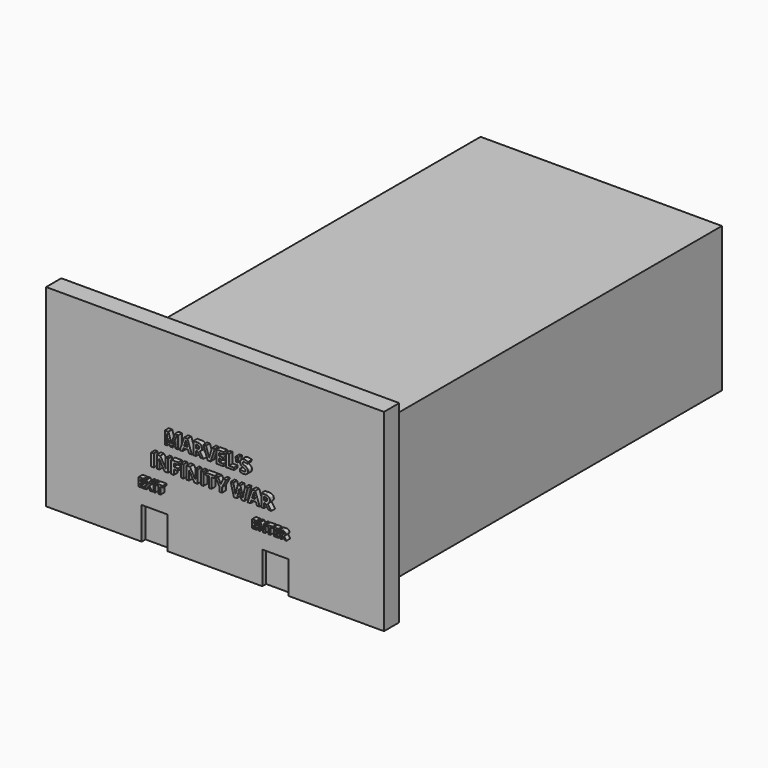
from build123d import *

# Parameters (mm, degrees)
F0_W          = 15240
F0_H          = 9144
F1_DEPTH      = 30480
F2_W          = 15240
F2_H          = 1203.030090332
F3_DEPTH      = 3048
F4_W          = 822.96
F4_H          = 2042.16
F5_DEPTH      = 304.8
F7_TEXT_SIZE  = 751.4417171478
F8_DEPTH      = 304.8
F9_TEXT_SIZE  = 701.0988429122
F10_DEPTH     = 304.8
F12_DEPTH     = 3048
F14_DEPTH     = 3048
F15_TEXT_SIZE = 1106.0376962026
F16_DEPTH     = 304.8


# Not quite as in the source:
# - Text() gives the source's letters only with a copy of the font that has no kerning and outlines rounded to 1/6400 em; it was checked with that copy


with BuildPart() as f1:
    # F0 (on Front) → F1 (new body)
    with BuildSketch(Plane.XZ):
        with Locations((7566.6301758587, 4516.3960119644)):
            Rectangle(F0_W, F0_H)
    extrude(amount=F1_DEPTH)

    # F2 (on face) → F3 (join)
    with BuildSketch(Plane.XY.offset(9088.3960119644)):
        with Locations((7566.6301758587, -29878.484954834)):
            Rectangle(F2_W, F2_H)
    extrude(amount=F3_DEPTH)

    # F4 (on face) → F5 (cut)
    with BuildSketch(Plane.XZ.offset(30480)):
        with Locations((3345.1501758587, 965.4760119644)):
            Rectangle(F4_W, F4_H)
        with Locations((4168.1101758587, 965.4760119644)):
            Rectangle(F4_W, F4_H)
        with Locations((10965.1501758587, 965.4760119644)):
            Rectangle(F4_W, F4_H)
        with Locations((11788.1101758587, 965.4760119644)):
            Rectangle(F4_W, F4_H)
    extrude(amount=-F5_DEPTH, mode=Mode.SUBTRACT)

    # F7 (on face) → F8 (join)
    with BuildSketch(Plane.XZ.offset(30480)):
        with Locations((2924.5324134827, 3148.3218669891)):
            Text('EXIT', F7_TEXT_SIZE, font='Open Sans', font_style=FontStyle.BOLD, text_align=(TextAlign.LEFT, TextAlign.BOTTOM))
    extrude(amount=F8_DEPTH)

    # F9 (on face) → F10 (join)
    with BuildSketch(Plane.XZ.offset(30480)):
        with Locations((10086.7914789268, 3166.4858793068)):
            Text('ENTER', F9_TEXT_SIZE, font='Open Sans', font_style=FontStyle.BOLD, text_align=(TextAlign.LEFT, TextAlign.BOTTOM))
    extrude(amount=F10_DEPTH)

    # F11 (on face) → F12 (join)
    with BuildSketch(Plane.YZ.offset(15186.6301758587)):
        Polygon((-29276.969909668, -55.6039880356), (-29276.969909668, 9088.3960119644), (-29276.969909668, 12136.3960119644), (-30480, 12136.3960119644), (-30480, -55.6039880356), align=None)
    extrude(amount=F12_DEPTH)

    # F13 (on face) → F14 (join)
    with BuildSketch(Plane(origin=(-53.3698241413, 0, 0), x_dir=(0, -1, 0), z_dir=(-1, 0, 0))):
        Polygon((29276.969909668, 12136.3960119644), (29276.969909668, 9088.3960119644), (29276.969909668, -55.6039880356), (30480, -55.6039880356), (30480, 12136.3960119644), align=None)
    extrude(amount=F14_DEPTH)

    # F15 (on face) → F16 (join)
    with BuildSketch(Plane.XZ.offset(30480)):
        with Locations((4538.9733174816, 6019.8884010315)):
            Text("MARVEL'S", F15_TEXT_SIZE, font='Open Sans', font_style=FontStyle.BOLD, text_align=(TextAlign.LEFT, TextAlign.BOTTOM))
        with Locations((3676.7823696136, 4515.677134196)):
            Text('INFINITY WAR', F15_TEXT_SIZE, font='Open Sans', font_style=FontStyle.BOLD, text_align=(TextAlign.LEFT, TextAlign.BOTTOM))
    extrude(amount=F16_DEPTH)


solid = f1.part
